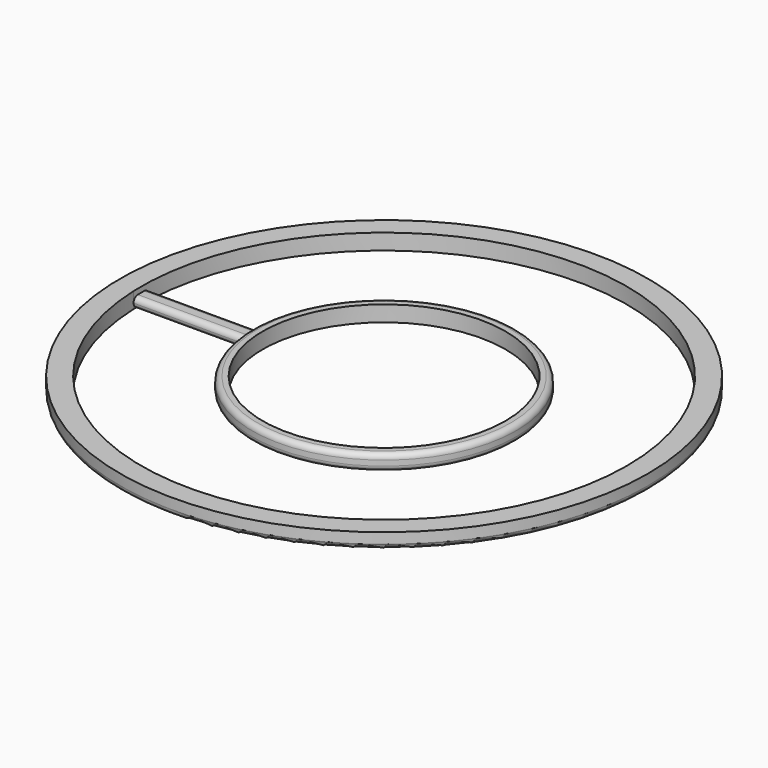
from build123d import *

# Parameters (mm, degrees)
F0_R     = 250
F1_DEPTH = 15
F0_R_2   = 115
F2_DEPTH = 10
F3_R     = 4.99999
F3_2_R   = 4.99999
F3_3_R   = 4.99999


# Not quite as in the source:
# - a fillet or chamfer is up to 0.001 mm smaller than in the source, because OpenCascade refuses the exact size


with BuildPart() as f1:
    # F0 (on Top) → F1 (new body)
    with BuildSketch(Plane.XY):
        Circle(F0_R)
        with BuildLine():
            ThreePointArc((-229.8105899104, -9.3323504552), (-229.9992492988, -0.5876410446), (-229.8552770118, 8.1579182297))
            ThreePointArc((-229.8552770118, 8.1579182297), (4.0796009175, 229.9638164067), (230, 0))
            ThreePointArc((230, 0), (4.667136199, -229.9526426021), (-229.8105899104, -9.3323504552))
        make_face(mode=Mode.SUBTRACT)
    extrude(amount=F1_DEPTH)

    # F3#2 (radius 5 in the source; OpenCascade refuses exactly that, so slightly less here)
    f3_2_edges = [f1.edges().sort_by_distance(p)[0] for p in [
        (-250, 0, 0),
    ]]
    fillet(f3_2_edges, radius=F3_2_R)


with BuildPart() as f1b:
    # F0 (on Top) → F1, piece 2 (new body)
    with BuildSketch(Plane.XY):
        with BuildLine():
            ThreePointArc((-124.6511421327, -9.3323504552), (4.6694343027, -124.9127550865), (125, 0))
            ThreePointArc((125, 0), (4.0811348629, 124.9333595891), (-124.7335094117, 8.1579182297))
            ThreePointArc((-124.7335094117, 8.1579182297), (-124.9986139169, -0.5886585218), (-124.6511421327, -9.3323504552))
        make_face()
        Circle(F0_R_2, mode=Mode.SUBTRACT)
    extrude(amount=F1_DEPTH)

    # F3#3 (radius 5 in the source; OpenCascade refuses exactly that, so slightly less here)
    f3_3_edges = [f1b.edges().sort_by_distance(p)[0] for p in [
        (-124.998614, -0.588659, 0),
        (-125, 0, 15),
    ]]
    fillet(f3_3_edges, radius=F3_3_R)


with BuildPart() as f2:
    # F0 (on Top) → F2 (new body)
    with BuildSketch(Plane.XY):
        with BuildLine():
            ThreePointArc((-124.6511421327, -9.3323504552), (-124.9986139169, -0.5886585218), (-124.7335094117, 8.1579182297))
            Line((-124.7335094117, 8.1579182297), (-229.8552770118, 8.1579182297))
            ThreePointArc((-229.8552770118, 8.1579182297), (-229.9992492988, -0.5876410446), (-229.8105899104, -9.3323504552))
            Line((-229.8105899104, -9.3323504552), (-124.6511421327, -9.3323504552))
        make_face()
    extrude(amount=F2_DEPTH)

    # F3 (radius 5 in the source; OpenCascade refuses exactly that, so slightly less here)
    f3_edges = [f2.edges().sort_by_distance(p)[0] for p in [
        (-177.294393, 8.157918, 0),
        (-177.230866, -9.33235, 0),
        (-177.294393, 8.157918, 10),
        (-177.230866, -9.33235, 10),
    ]]
    fillet(f3_edges, radius=F3_R)


solid = Compound([f1.part, f1b.part, f2.part])
